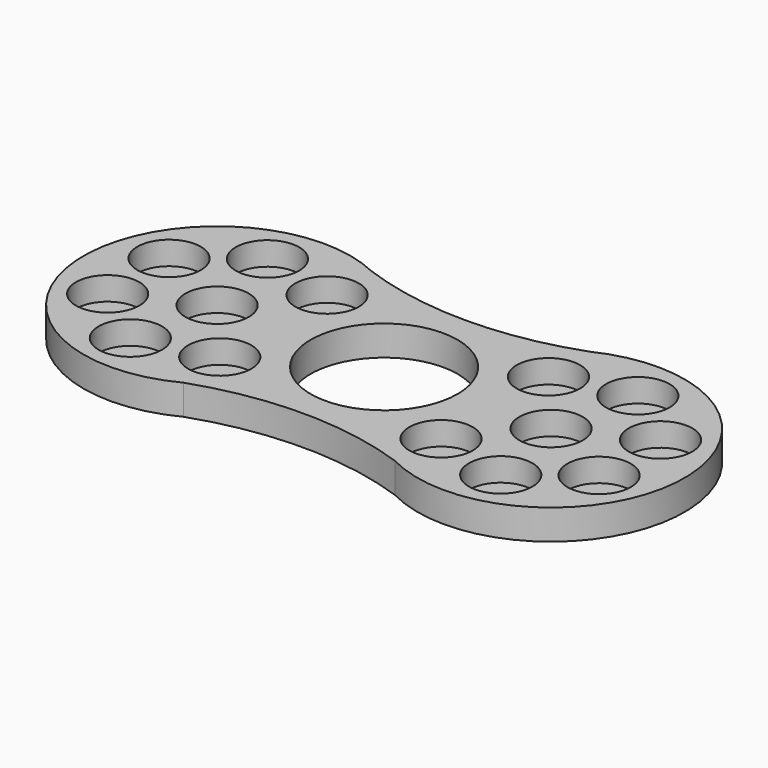
from build123d import *

# Parameters (mm, degrees)
F0_R     = 4.75
F0_R_2   = 11
F1_DEPTH = 4.5
F2_DEPTH = 1


# Not quite as in the source:
# - a feature names something its author has since deleted; it is built from what else it names


with BuildPart() as f1:
    # F0 (on Top) → F1 (new body)
    with BuildSketch(Plane.XY):
        with BuildLine():
            ThreePointArc((-15.8212677669, -17.7693802535), (0, -15.0870091218), (15.8212677669, -17.7693802535))
            ThreePointArc((15.8212677669, -17.7693802535), (44.9980398453, -0.2800041916), (16.3223672692, 18.019397609))
            ThreePointArc((16.3223672692, 18.019397609), (0, 15.1589625906), (-16.3223672692, 18.019397609))
            ThreePointArc((-16.3223672692, 18.019397609), (-44.9980398453, -0.2800041916), (-15.8212677669, -17.7693802535))
        make_face()
        with Locations((-27.7271234226, -12.8301069662)):
            Circle(F0_R, mode=Mode.SUBTRACT)
        with Locations((-16.5687225704, -10.0480051668)):
            Circle(F0_R, mode=Mode.SUBTRACT)
        with Locations((-36.7892470891, -5.75)):
            Circle(F0_R, mode=Mode.SUBTRACT)
        with Locations((16.5687225704, -10.0480051668)):
            Circle(F0_R, mode=Mode.SUBTRACT)
        with Locations((27.7271234226, -12.8301069662)):
            Circle(F0_R, mode=Mode.SUBTRACT)
        with Locations((36.7892470891, -5.75)):
            Circle(F0_R, mode=Mode.SUBTRACT)
        with Locations((-25, 0)):
            Circle(F0_R, mode=Mode.SUBTRACT)
        with Locations((-36.7892470891, 5.75)):
            Circle(F0_R, mode=Mode.SUBTRACT)
        with Locations((-27.7271234226, 12.8301069662)):
            Circle(F0_R, mode=Mode.SUBTRACT)
        with Locations((-16.5687225704, 10.0480051668)):
            Circle(F0_R, mode=Mode.SUBTRACT)
        Circle(F0_R_2, mode=Mode.SUBTRACT)
        with Locations((25, 0)):
            Circle(F0_R, mode=Mode.SUBTRACT)
        with Locations((36.7892470891, 5.75)):
            Circle(F0_R, mode=Mode.SUBTRACT)
        with Locations((16.5687225704, 10.0480051668)):
            Circle(F0_R, mode=Mode.SUBTRACT)
        with Locations((27.7271234226, 12.8301069662)):
            Circle(F0_R, mode=Mode.SUBTRACT)
    extrude(amount=F1_DEPTH)

    # F0 (on Top) → F2 (join)
    with BuildSketch(Plane.XY):
        with Locations((-25, 0)):
            Circle(F0_R)
        with Locations((25, 0)):
            Circle(F0_R)
        with Locations((-16.5687225704, 10.0480051668)):
            Circle(F0_R)
        with Locations((-27.7271234226, 12.8301069662)):
            Circle(F0_R)
        with Locations((-36.7892470891, 5.75)):
            Circle(F0_R)
        with Locations((-36.7892470891, -5.75)):
            Circle(F0_R)
        with Locations((-27.7271234226, -12.8301069662)):
            Circle(F0_R)
        with Locations((-16.5687225704, -10.0480051668)):
            Circle(F0_R)
        with Locations((16.5687225704, 10.0480051668)):
            Circle(F0_R)
        with Locations((27.7271234226, 12.8301069662)):
            Circle(F0_R)
        with Locations((36.7892470891, 5.75)):
            Circle(F0_R)
        with Locations((36.7892470891, -5.75)):
            Circle(F0_R)
        with Locations((27.7271234226, -12.8301069662)):
            Circle(F0_R)
        with Locations((16.5687225704, -10.0480051668)):
            Circle(F0_R)
    extrude(amount=F2_DEPTH)


solid = f1.part
